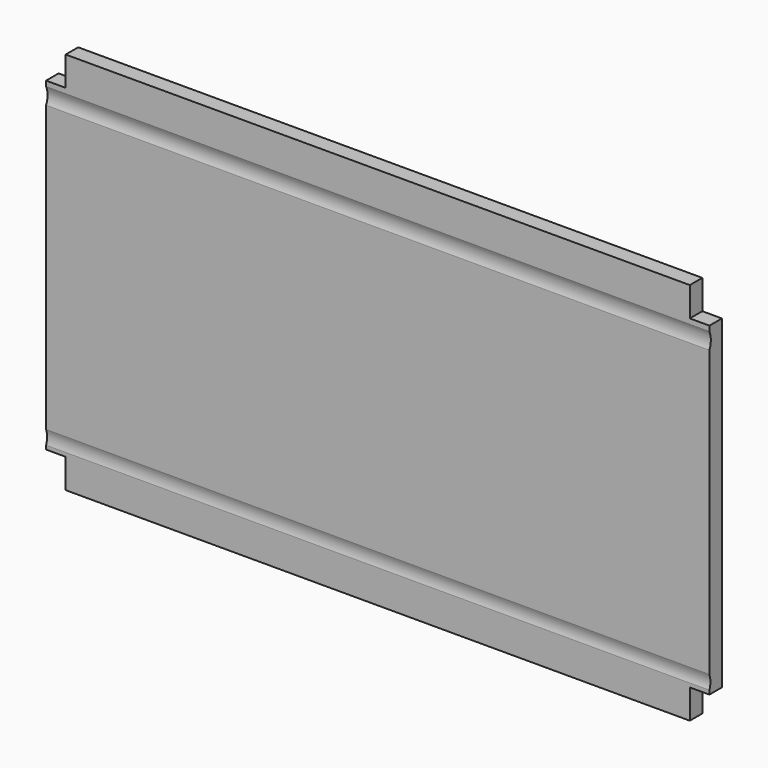
from build123d import *

# Parameters (mm, degrees)
F0_W      = 1695
F0_H      = 980
F1_DEPTH  = 40
F2_R      = 50
F3_DEPTH  = 1695.001
F6_W      = 40
F6_H      = 75
F7_DEPTH  = 50
F8_W      = 40
F8_H      = 75
F9_DEPTH  = 50
F10_SCALE = 0.05


# Not quite as in the source:
# - a feature of the source that left no trace in its solid (it failed there, or was rolled back) is left out


with BuildPart() as f1:
    # F0 (on Front) → F1 (new body)
    with BuildSketch(Plane.XZ):
        with Locations((847.5, -490)):
            Rectangle(F0_W, F0_H)
    extrude(amount=F1_DEPTH)

    # F2 (on face) → F3 (cut, through all)
    with BuildSketch(Plane(origin=(0, 0, 0), x_dir=(0, -1, 0), z_dir=(-1, 0, 0))):
        with Locations((85.3642523289, -109.1325581074)):
            Circle(F2_R)
        with Locations((86.7706388235, -877.3503899574)):
            Circle(F2_R)
    extrude(amount=-F3_DEPTH, mode=Mode.SUBTRACT)

    # F6 (on face) → F7 (cut)
    with BuildSketch(Plane(origin=(0, 0, 0), x_dir=(0, -1, 0), z_dir=(-1, 0, 0))):
        with Locations((20, -37.5)):
            Rectangle(F6_W, F6_H)
        with Locations((20, -942.5)):
            Rectangle(F6_W, F6_H)
    extrude(amount=-F7_DEPTH, mode=Mode.SUBTRACT)

    # F8 (on face) → F9 (cut)
    with BuildSketch(Plane.YZ.offset(1695)):
        with Locations((-20, -37.5)):
            Rectangle(F8_W, F8_H)
        with Locations((-20, -942.5)):
            Rectangle(F8_W, F8_H)
    extrude(amount=-F9_DEPTH, mode=Mode.SUBTRACT)


with BuildPart() as f1_1:
    # F10: moved
    add(f1.part.scale(F10_SCALE))


solid = f1_1.part
